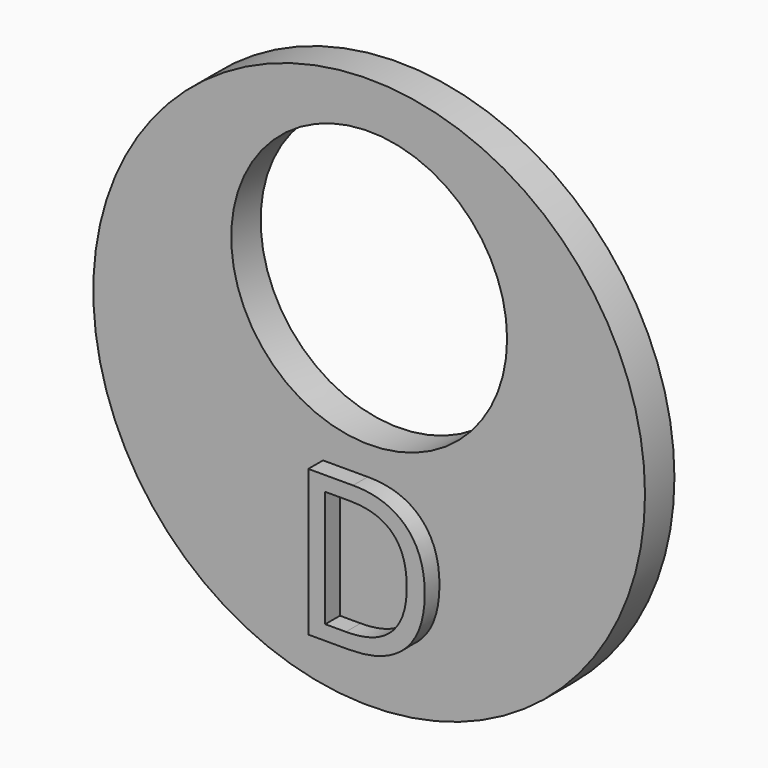
from build123d import *

# Parameters (mm, degrees)
F0_R         = 15
F0_R_2       = 7.5
F1_DEPTH     = 2
F2_TEXT_SIZE = 11.1111111111
F3_DEPTH     = 1


# Not quite as in the source:
# - Text() gives the source's letters only with a copy of the font that has no kerning and outlines rounded to 1/6400 em; it was checked with that copy


with BuildPart() as f1:
    # F0 (on Front) → F1 (new body)
    with BuildSketch(Plane.XZ):
        Circle(F0_R)
        with Locations((0, 5)):
            Circle(F0_R_2, mode=Mode.SUBTRACT)
    extrude(amount=F1_DEPTH)

    # F2 (on face) → F3 (join)
    with BuildSketch(Plane.XZ.offset(2)):
        with Locations((-3.5999998973, -12)):
            Text('D', F2_TEXT_SIZE, font='Open Sans', text_align=(TextAlign.LEFT, TextAlign.BOTTOM))
    extrude(amount=F3_DEPTH)


solid = f1.part
